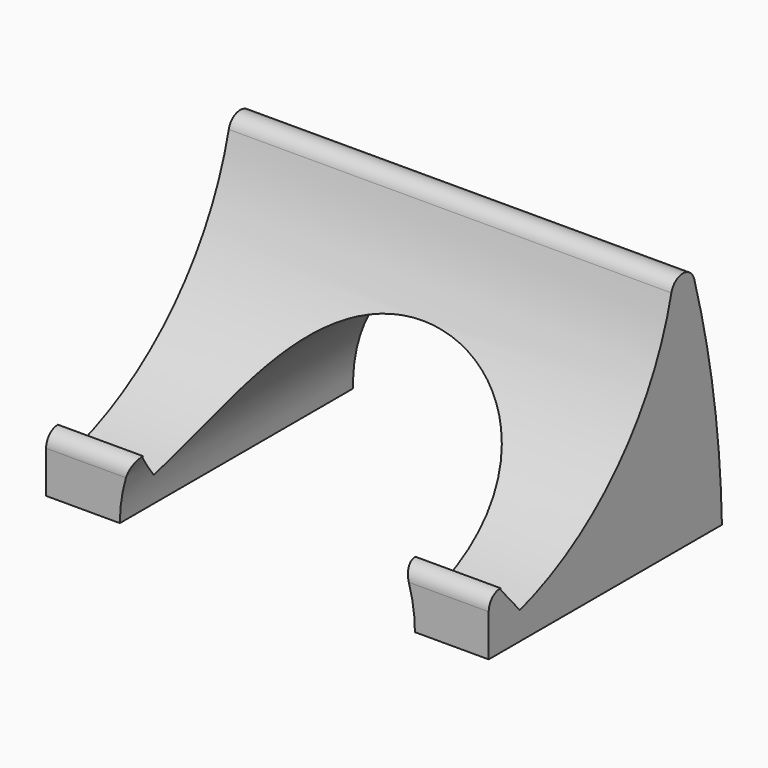
from build123d import *

# Parameters (mm, degrees)
F0_W        = 19.1873764305
F0_H        = 101.6
F1_DEPTH    = 76.2
F3_DEPTH    = 67.31
F4_T1_DEPTH = 697.6501262753
F5_R        = 5.07999
F6_R        = 5.08


# Not quite as in the source:
# - a fillet or chamfer that OpenCascade refuses, or shapes differently, is made with other operations: its cross-section is extruded or revolved along the edge and cut away or added
# - a fillet or chamfer is up to 0.001 mm smaller than in the source, because OpenCascade refuses the exact size


with BuildPart() as f1:
    # F0 (on Right) → F1 (new body, symmetric)
    with BuildSketch(Plane.YZ):
        with BuildLine():
            Line((-28.6442058678, -4.364277937), (-36.9899753063, 5.2085028753))
            Line((-36.9899753063, 5.2085028753), (-36.9899753063, -13.8414971247))
            Line((-36.9899753063, -13.8414971247), (39.2100246937, -13.8414971247))
            Line((39.2100246937, -13.8414971247), (39.2100246937, 87.7585028753))
            ThreePointArc((39.2100246937, 87.7585028753), (20.4155377225, 30.5509785676), (-28.6442058678, -4.364277937))
        make_face()
        Polygon((-36.9899753063, -13.8414971247), (-36.9899753063, 5.2085028753), (-36.9899753063, 5.6934356689), (-42.0699753063, 5.6934356689), (-42.0699753063, -13.8414971247), align=None)
        with Locations((48.803712909, 36.9585028753)):
            Rectangle(F0_W, F0_H)
    extrude(amount=F1_DEPTH, both=True)

    # F2 (on Front) → F3 (cut, symmetric)
    with BuildSketch(Plane.XZ):
        with BuildLine():
            ThreePointArc((50.7993000876, -14.1734545694), (0.1539604747, 36.9344649658), (-50.8002333049, -13.8655350342))
            Line((-50.8002333049, -13.8655350342), (50.7993000876, -14.1734545694))
        make_face()
    extrude(amount=F3_DEPTH, both=True, mode=Mode.SUBTRACT)

    # F4: fillet of radius 319.4825375631 on 1 edges, made by hand

    # F4_s2 → F4_t1 (cut)
    with BuildSketch(Plane.YZ.offset(-348.8250631377)):
        with BuildLine():
            ThreePointArc((39.2100246937, 87.7585028753), (53.5639950587, 34.0710629609), (58.3974011242, -21.2915223798))
            Line((58.3974011242, -21.2915223798), (64.7870518755, -21.2915223798))
            Line((64.7870518755, -21.2915223798), (64.7870518755, 87.7585028753))
            Line((64.7870518755, 87.7585028753), (58.3974011242, 94.1481536266))
            ThreePointArc((58.3974011242, 94.1481536266), (48.803712909, 94.1481536266), (45.2159279163, 89.9395033804))
            Line((45.2159279163, 89.9395033804), (39.2100246937, 87.7585028753))
        make_face()
    extrude(amount=F4_T1_DEPTH, mode=Mode.SUBTRACT)

    # F5 (radius 5.08 in the source; OpenCascade refuses exactly that, so slightly less here)
    f5_edges = [f1.edges().sort_by_distance(p)[0] for p in [
        (-61.542005, -42.069975, 5.693436),
        (61.542005, -42.069975, 5.693436),
    ]]
    fillet(f5_edges, radius=F5_R)

    # F6
    f6_edges = [f1.edges().sort_by_distance(p)[0] for p in [
        (0, 39.210025, 87.758503),
    ]]
    fillet(f6_edges, radius=F6_R)


solid = f1.part
